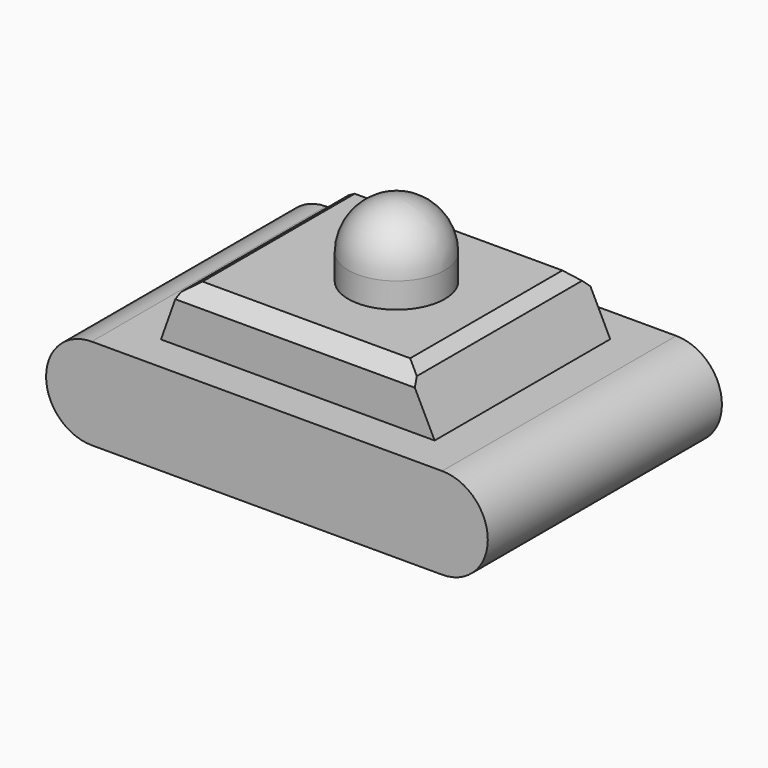
from build123d import *

# Parameters (mm, degrees)
F1_DEPTH    = 50
F2_DEPTH    = 37.5
F4_T1_DEPTH = 103.3030187921
F4_T3_DEPTH = 91.394543157
F4_T5_DEPTH = 93.4430330881


# Not quite as in the source:
# - a fillet or chamfer that OpenCascade refuses, or shapes differently, is made with other operations: its cross-section is extruded or revolved along the edge and cut away or added


with BuildPart() as f1:
    # F0 (on Front) → F1 (new body, symmetric)
    with BuildSketch(Plane.XZ):
        with BuildLine():
            Line((-59.8632097244, -15.5979888514), (59.8632097244, -15.5979888514))
            ThreePointArc((59.8632097244, -15.5979888514), (75.4611985758, 0), (59.8632097244, 15.5979888514))
            Line((59.8632097244, 15.5979888514), (47.2922846675, 15.5979888514))
            Line((47.2922846675, 15.5979888514), (-46.2039783597, 15.5979888514))
            Line((-46.2039783597, 15.5979888514), (-59.8632097244, 15.5979888514))
            ThreePointArc((-59.8632097244, 15.5979888514), (-75.4611985758, 0), (-59.8632097244, -15.5979888514))
        make_face()
    extrude(amount=F1_DEPTH, both=True)

    # F0 (on Front) → F2 (join, symmetric)
    with BuildSketch(Plane.XZ):
        Polygon((-46.2039783597, 15.5979888514), (47.2922846675, 15.5979888514), (38.0605123937, 34.2928767204), (20.7754876465, 34.2928767204), (4.2761466466, 34.2928767204), (-12.2231943533, 34.2928767204), (-39.5256765187, 34.2928767204), align=None)
    extrude(amount=F2_DEPTH, both=True)

    # F0 (on Front) → F3 (revolve)
    with BuildSketch(Plane.XZ):
        with BuildLine():
            Line((4.2761466466, 34.2928767204), (20.7754876465, 34.2928767204))
            Line((20.7754876465, 34.2928767204), (20.7754876465, 42.9353863001))
            ThreePointArc((20.7754876465, 42.9353863001), (15.9429425527, 54.6021822062), (4.2761466466, 59.4347273))
            Line((4.2761466466, 59.4347273), (4.2761466466, 42.9353863001))
            Line((4.2761466466, 42.9353863001), (4.2761466466, 34.2928767204))
        make_face()
    revolve(axis=Axis((4.2761466466, 0, 51.1850568), (0, 0, 1)))

    # F4: chamfer of 5 on 4 edges, made by hand

    # F4_s2 → F4_t1 (cut)
    with BuildSketch(Plane.YZ.offset(-52.3840914585)):
        Polygon((-37.5, 29.2928767204), (-32.5, 34.2928767204), (-37.5, 34.2928767204), align=None)
        Polygon((37.5, 29.2928767204), (32.5, 34.2928767204), (37.5, 34.2928767204), align=None)
    extrude(amount=F4_T1_DEPTH, mode=Mode.SUBTRACT)

    # F4_s4 → F4_t3 (cut)
    with BuildSketch(Plane.XZ.offset(-45.6972715785)):
        Polygon((39.4363488807, 31.506726013), (34.9531724053, 34.2928767204), (38.0605123937, 34.2928767204), align=None)
    extrude(amount=F4_T3_DEPTH, mode=Mode.SUBTRACT)

    # F4_s6 → F4_t5 (cut)
    with BuildSketch(Plane.XZ.offset(-46.7215165441)):
        Polygon((-40.7109421413, 30.9749063085), (-36.0023567418, 34.2928767204), (-39.5256765187, 34.2928767204), align=None)
    extrude(amount=F4_T5_DEPTH, mode=Mode.SUBTRACT)


solid = f1.part
